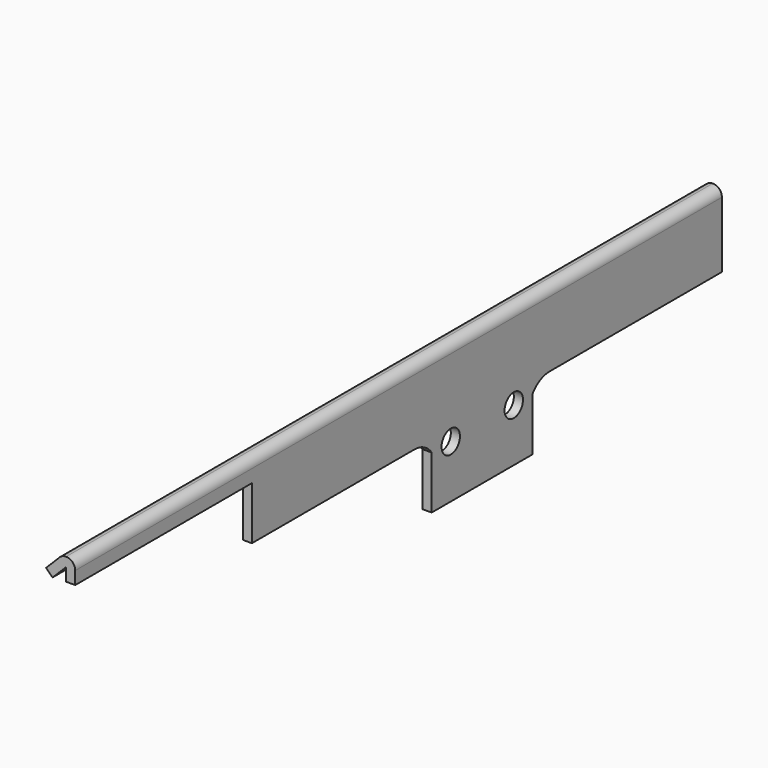
from build123d import *

# Parameters (mm, degrees)
F0_W      = 139.446
F0_H      = 24.0284
F1_DEPTH  = 1.5748
F2_R      = 2.5273
F2_R_2    = 1.9812
F3_DEPTH  = 25.4
F4_W      = 76.8604
F4_H      = 9.1186
F4_W_2    = 40.894
F5_DEPTH  = 25.4
F7_DEPTH  = 25.4
F9_DEPTH  = 139.447
F10_DEPTH = 139.446
F11_R     = 2.5273
F12_DEPTH = 25.4
F14_DEPTH = 1.5748
F15_DEPTH = 25.4


# Not quite as in the source:
# - ends of sketch curves that miss each other by under 0.0002 mm in the source are joined


with BuildPart() as f1:
    # F0 (on Right) → F1 (new body)
    with BuildSketch(Plane.YZ):
        with Locations((69.723, 12.0142)):
            Rectangle(F0_W, F0_H)
    extrude(amount=F1_DEPTH)

    # F2 (on face) → F3 (cut)
    with BuildSketch(Plane.YZ.offset(1.5748)):
        with Locations((7.9502, 14.6812)):
            Circle(F2_R)
        with Locations((80.9752, 9.1186)):
            Circle(F2_R_2)
        with Locations((94.5642, 9.1186)):
            Circle(F2_R_2)
    extrude(amount=-F3_DEPTH, mode=Mode.SUBTRACT)

    # F4 (on face) → F5 (cut)
    with BuildSketch(Plane.YZ.offset(1.5748)):
        with Locations((38.4302, 4.5593)):
            Rectangle(F4_W, F4_H)
        with Locations((118.999, 4.5593)):
            Rectangle(F4_W_2, F4_H)
    extrude(amount=-F5_DEPTH, mode=Mode.SUBTRACT)

    # F6 (on face) → F7 (cut)
    with BuildSketch(Plane.YZ.offset(1.5748)):
        with BuildLine():
            ThreePointArc((102.3057040906, 11.0998), (104.4279345117, 10.5741090514), (106.0594081813, 9.1186))
            Line((106.0594081813, 9.1186), (139.446, 9.1186))
            Line((139.446, 9.1186), (139.446, 11.0998))
            Line((139.446, 11.0998), (102.3057040906, 11.0998))
        make_face()
        with BuildLine():
            Line((98.552, 9.1186), (106.0594081813, 9.1186))
            ThreePointArc((106.0594081813, 9.1186), (104.4279345117, 10.5741090514), (102.3057040906, 11.0998))
            ThreePointArc((102.3057040906, 11.0998), (100.1834736696, 10.5741090514), (98.552, 9.1186))
        make_face()
        with BuildLine():
            ThreePointArc((25.0643040906, 9.1186), (23.4328304559, 10.574109033), (21.3106000788, 11.0998))
            ThreePointArc((21.3106000788, 11.0998), (19.1883696138, 10.5741090698), (17.5568959094, 9.1186))
            Line((17.5568959094, 9.1186), (25.0643040906, 9.1186))
        make_face()
        with BuildLine():
            ThreePointArc((69.3529918187, 9.1186), (70.9844654883, 10.5741090514), (73.1066959094, 11.0998))
            Line((73.1066959094, 11.0998), (21.3106000788, 11.0998))
            ThreePointArc((21.3106000788, 11.0998), (23.4328304559, 10.574109033), (25.0643040906, 9.1186))
            Line((25.0643040906, 9.1186), (69.3529918187, 9.1186))
        make_face()
        with BuildLine():
            ThreePointArc((76.8604, 9.1186), (75.2289263304, 10.5741090514), (73.1066959094, 11.0998))
            ThreePointArc((73.1066959094, 11.0998), (70.9844654883, 10.5741090514), (69.3529918187, 9.1186))
            Line((69.3529918187, 9.1186), (76.8604, 9.1186))
        make_face()
    extrude(amount=-F7_DEPTH, mode=Mode.SUBTRACT)

    # F8 (on face) → F9 (cut, through all)
    with BuildSketch(Plane.XZ):
        with BuildLine():
            Line((1.5748, 24.0284), (0, 24.0284))
            ThreePointArc((0, 24.0284), (1.1139794542, 23.562560882), (1.5748, 22.4465026135))
            Line((1.5748, 22.4465026135), (1.5748, 24.0284))
        make_face()
    extrude(amount=-F9_DEPTH, mode=Mode.SUBTRACT)

    # F8 (on face) → F10 (join)
    with BuildSketch(Plane.XZ):
        with BuildLine():
            Line((0, 24.0284), (0, 22.4536))
            Line((0, 22.4536), (0, 22.4465026135))
            Line((0, 22.4465026135), (1.5748, 22.4465026135))
            ThreePointArc((1.5748, 22.4465026135), (1.1139794542, 23.562560882), (0, 24.0284))
        make_face()
        with BuildLine():
            Line((-1.2264893587, 23.4542141594), (-0.0070973865, 22.4465026135))
            Line((-0.0070973865, 22.4465026135), (0, 22.4536))
            Line((0, 22.4536), (0, 24.0284))
            ThreePointArc((0, 24.0284), (-0.6777928151, 23.8791808689), (-1.2264893587, 23.4542141594))
        make_face()
        Polygon((-3.4544, 21.226303518), (-2.340848241, 20.112751759), (-0.0070973865, 22.4465026135), (-1.2264893587, 23.4542141594), align=None)
    extrude(amount=-F10_DEPTH)

    # F11 (on face) → F12 (cut)
    with BuildSketch(Plane(origin=(0, 0, 0), x_dir=(0, -1, 0), z_dir=(-1, 0, 0))):
        with BuildLine():
            Line((-17.5568959094, 9.1186), (0, 9.1186))
            Line((0, 9.1186), (0, 20.2311))
            Line((0, 20.2311), (-38.1, 20.2311))
            Line((-38.1, 20.2311), (-38.1, 11.0998))
            Line((-38.1, 11.0998), (-21.3106000788, 11.0998))
            ThreePointArc((-21.3106000788, 11.0998), (-19.1883696138, 10.5741090698), (-17.5568959094, 9.1186))
        make_face()
        with Locations((-7.9502, 14.6812)):
            Circle(F11_R, mode=Mode.SUBTRACT)
    extrude(amount=-F12_DEPTH, mode=Mode.SUBTRACT)


with BuildPart() as f14:
    # F13 (on Right) → F14 (new body, through all)
    with BuildSketch(Plane.YZ):
        with BuildLine():
            Line((38.1, 20.2311), (0, 20.2311))
            Line((0, 20.2311), (0, 0))
            Line((0, 0), (16.764, 0))
            Line((16.764, 0), (16.764, 6.5532))
            ThreePointArc((16.764, 6.5532), (18.0956683087, 9.7681316913), (21.3106, 11.0998))
            Line((21.3106, 11.0998), (38.1, 11.0998))
            Line((38.1, 11.0998), (38.1, 20.2311))
        make_face()
    extrude(amount=F14_DEPTH)

    # F2 (on face) → F15 (cut)
    with BuildSketch(Plane.YZ.offset(1.5748)):
        with Locations((7.9502, 14.6812)):
            Circle(F2_R)
    extrude(amount=-F15_DEPTH, mode=Mode.SUBTRACT)


solid = f1.part
